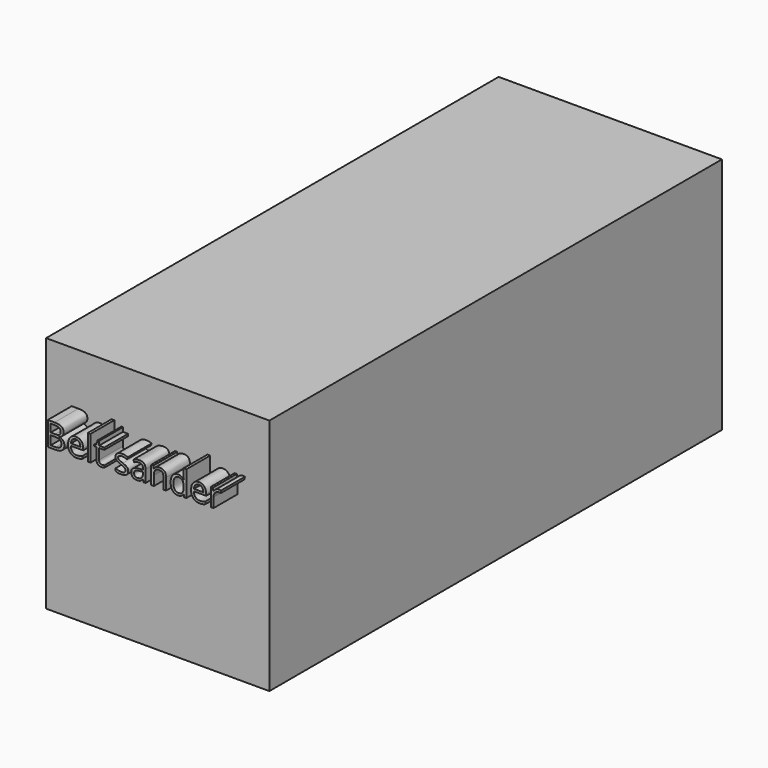
from build123d import *

# Parameters (mm, degrees)
F0_W         = 190.5
F0_H         = 203.2
F1_DEPTH     = 482.6
F2_TEXT_SIZE = 28.4618751641
F3_DEPTH     = 25.4


# Not quite as in the source:
# - Text() gives the source's letters only with a copy of the font that has no kerning and outlines rounded to 1/6400 em; it was checked with that copy


with BuildPart() as f1:
    # F0 (on Front) → F1 (new body)
    with BuildSketch(Plane.XZ):
        Rectangle(F0_W, F0_H)
    extrude(amount=F1_DEPTH)

    # F2 (on face) → F3 (join)
    with BuildSketch(Plane.XZ.offset(482.6)):
        with Locations((-76.2, 37.264749925)):
            Text('Belt sander', F2_TEXT_SIZE, font='Open Sans', text_align=(TextAlign.LEFT, TextAlign.BOTTOM))
    extrude(amount=F3_DEPTH)


solid = f1.part
